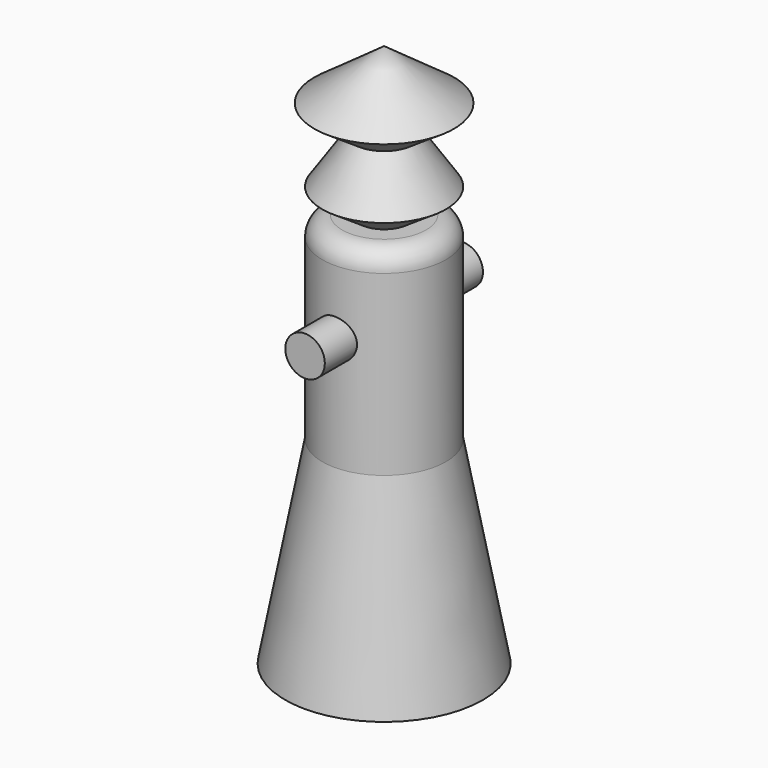
from build123d import *

# Parameters (mm, degrees)
F0_R     = 25.4
F2_R     = 15.875
F4_R     = 15.875
F5_DEPTH = 50.8
F6_R     = 5.08
F7_DEPTH = 25.4
F8_DEPTH = 50.8
F9_R     = 5.08


with BuildPart() as f3:
    # F0 (on Top) → F3 section 0
    with BuildSketch(Plane.XY):
        Circle(F0_R)
    # F2 (on offset) → F3 section 1
    with BuildSketch(Plane.XY.offset(50.8)):
        Circle(F2_R)
    loft()

    # F4 (on face) → F5 (join)
    with BuildSketch(Plane.XY.offset(50.8)):
        Circle(F4_R)
    extrude(amount=F5_DEPTH)

    # F6 (on Front) → F7 (join)
    with BuildSketch(Plane.XZ):
        with Locations((0, 79.9094587564)):
            Circle(F6_R)
    extrude(amount=F7_DEPTH)

    # F8 (add): a face of the model
    f8_faces = [f3.faces().sort_by_distance(p)[0] for p in [
        (0, -25.4, 79.9094587564),
    ]]
    extrude(f8_faces, amount=-F8_DEPTH)

    # F9
    f9_edges = [f3.edges().sort_by_distance(p)[0] for p in [
        (-15.875, 0, 101.6),
    ]]
    fillet(f9_edges, radius=F9_R)

    # F10 (on Front) → F11 (revolve)
    with BuildSketch(Plane.XZ):
        Polygon((-15.8836290712, 107.9245372937), (0, 97.2370281816), (0, 139.7015303373), (-17.9440863431, 126.805588603), (-7.7806902118, 119.9670135975), align=None)
    revolve(axis=Axis((0, 0, 69.8507651687), (0, 0, 1)))


solid = f3.part
